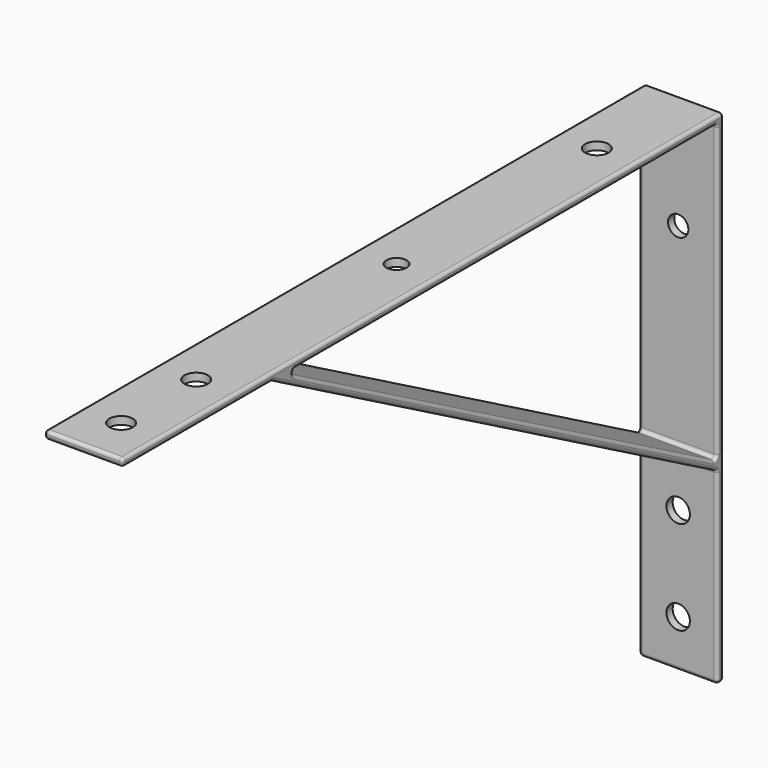
from build123d import *

# Parameters (mm, degrees)
F1_DEPTH = 31.75
F3_R     = 1.27
F4_R     = 4.7625
F4_R_2   = 4.1275
F5_DEPTH = 3.175
F6_R     = 4.7625
F6_R_2   = 4.1275
F7_DEPTH = 3.175


# Not quite as in the source:
# - a feature of the source that left no trace in its solid (it failed there, or was rolled back) is left out


with BuildPart() as f1:
    # F0 (on Right) → F1 (new body)
    with BuildSketch(Plane.YZ):
        Polygon((0, 203.2), (-304.8, 203.2), (-304.8, 200.025), (-228.6, 200.025), (-3.175, 76.2), (-3.175, 0), (0, 0), align=None)
        Polygon((-222.0052667175, 200.025), (-3.175, 200.025), (-3.175, 79.822459127), align=None, mode=Mode.SUBTRACT)
    extrude(amount=F1_DEPTH)

    # F3
    f3_edges = [f1.edges().sort_by_distance(p)[0] for p in [
        (15.875, -3.175, 79.822459),
        (15.875, -222.005267, 200.025),
        (15.875, -3.175, 200.025),
        (15.875, 0, 203.2),
        (15.875, -304.8, 203.2),
        (0, -152.4, 203.2),
        (31.75, -152.4, 203.2),
        (15.875, -304.8, 200.025),
        (0, -304.8, 201.6125),
        (31.75, -304.8, 201.6125),
        (0, -112.590133, 200.025),
        (31.75, -112.590133, 200.025),
        (15.875, 0, 0),
        (0, 0, 101.6),
        (31.75, 0, 101.6),
        (15.875, -3.175, 0),
        (0, -1.5875, 0),
        (31.75, -1.5875, 0),
        (15.875, -228.6, 200.025),
        (0, -266.7, 200.025),
        (31.75, -266.7, 200.025),
        (15.875, -3.175, 76.2),
        (0, -115.8875, 138.1125),
        (31.75, -115.8875, 138.1125),
        (0, -3.175, 38.1),
        (31.75, -3.175, 38.1),
        (0, -112.590133, 139.92373),
        (31.75, -112.590133, 139.92373),
        (0, -3.175, 139.92373),
        (31.75, -3.175, 139.92373),
    ]]
    fillet(f3_edges, radius=F3_R)

    # F4 (on face) → F5 (cut, through all)
    with BuildSketch(Plane(origin=(0, 0, 200.025), x_dir=(1, 0, 0), z_dir=(0, 0, -1))):
        with Locations((15.875, 285.75)):
            Circle(F4_R)
        with Locations((15.875, 247.65)):
            Circle(F4_R)
        with Locations((15.875, 146.05)):
            Circle(F4_R_2)
        with Locations((15.875, 44.45)):
            Circle(F4_R)
    extrude(amount=-F5_DEPTH, mode=Mode.SUBTRACT)

    # F6 (on face) → F7 (cut, through all)
    with BuildSketch(Plane.XZ.offset(3.175)):
        with Locations((15.875, 57.15)):
            Circle(F6_R)
        with Locations((15.875, 19.05)):
            Circle(F6_R)
        with Locations((15.875, 158.75)):
            Circle(F6_R_2)
    extrude(amount=-F7_DEPTH, mode=Mode.SUBTRACT)


solid = f1.part
